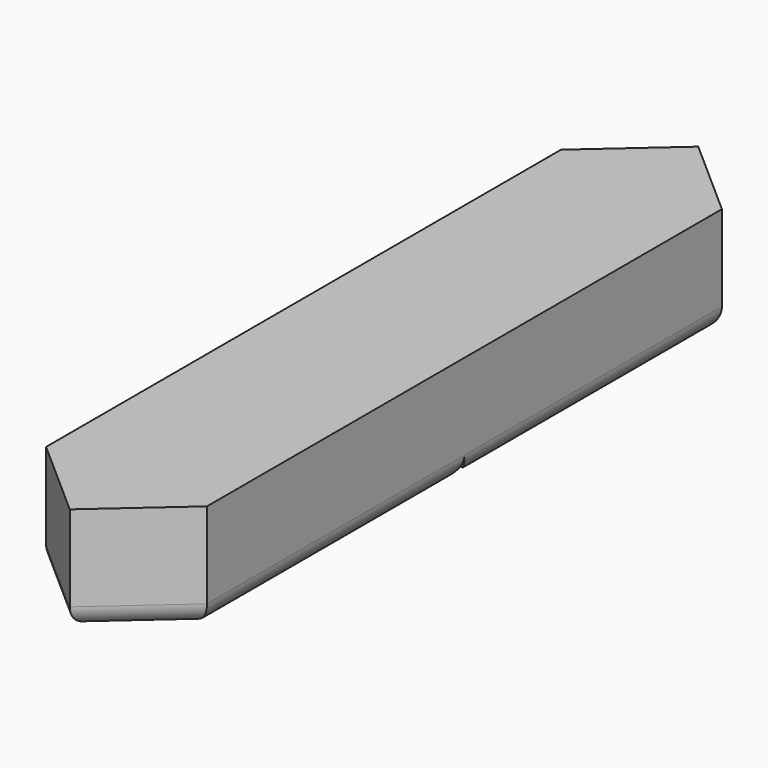
from build123d import *

# Parameters (mm, degrees)
F1_DEPTH    = 25.4
F0_W        = 38.1
F0_H        = 76.2
F2_DEPTH    = 25.4
F3_T        = -2.54
F4_T1_DEPTH = 101.6
F4_T3_DEPTH = 50.8
F4_T5_DEPTH = 50.8
F4_T7_DEPTH = 63.5


# Not quite as in the source:
# - a fillet or chamfer that OpenCascade refuses, or shapes differently, is made with other operations: its cross-section is extruded or revolved along the edge and cut away or added


with BuildPart() as f1:
    # F0 (on Top) → F1 (new body)
    with BuildSketch(Plane.XY):
        Polygon((25.0072174214, -22.3877525396), (-13.0927825786, -22.3877525396), (5.9572174214, -39.1882733649), align=None)
    extrude(amount=F1_DEPTH)

    # F0 (on Top) → F2 (join)
    with BuildSketch(Plane.XY):
        with Locations((5.9572174214, 15.7122474604)):
            Rectangle(F0_W, F0_H)
    extrude(amount=F2_DEPTH)

    # F3
    f3_openings = [f1.faces().sort_by_distance(p)[0] for p in [
        (5.957217, 11.373102, 0),
    ]]
    offset(amount=F3_T, openings=f3_openings)

    # F4: fillet of radius 5.08 on 5 edges, made by hand

    # F4_s2 → F4_t1 (cut)
    with BuildSketch(Plane.XZ.offset(-66.5122474604)):
        with BuildLine():
            ThreePointArc((25.0072174214, 5.08), (23.5193198698, 1.4878975516), (19.9272174214, 0))
            Line((19.9272174214, 0), (25.0072174214, 0))
            Line((25.0072174214, 0), (25.0072174214, 5.08))
        make_face()
        with BuildLine():
            ThreePointArc((-13.0927825786, 5.08), (-11.604885027, 1.4878975516), (-8.0127825786, 0))
            Line((-8.0127825786, 0), (-13.0927825786, 0))
            Line((-13.0927825786, 0), (-13.0927825786, 5.08))
        make_face()
    extrude(amount=F4_T1_DEPTH, mode=Mode.SUBTRACT)

    # F4_s4 → F4_t3 (cut)
    with BuildSketch(Plane(origin=(-25.6145200068, -22.5898832967, 0), x_dir=(0, 0, 1), z_dir=(0.75, 0.6614378278, 0))):
        with BuildLine():
            ThreePointArc((5.08, 33.3315339744), (1.4878975516, 31.8436364228), (0, 28.2515339744))
            Line((0, 28.2515339744), (0, 33.3315339744))
            Line((0, 33.3315339744), (5.08, 33.3315339744))
        make_face()
    extrude(amount=F4_T3_DEPTH, mode=Mode.SUBTRACT)

    # F4_s6 → F4_t5 (cut)
    with BuildSketch(Plane(origin=(-5.7836103942, 5.1006649277, 0), x_dir=(0, 0, 1), z_dir=(0.75, -0.6614378278, 0))):
        with BuildLine():
            ThreePointArc((5.08, 25.4508760729), (1.4878975516, 23.9629785214), (0, 20.3708760729))
            Line((0, 20.3708760729), (0, 25.4508760729))
            Line((0, 25.4508760729), (5.08, 25.4508760729))
        make_face()
    extrude(amount=F4_T5_DEPTH, mode=Mode.SUBTRACT)

    # F4_s8 → F4_t7 (cut)
    with BuildSketch(Plane.YZ.offset(-25.7927825786)):
        with BuildLine():
            ThreePointArc((53.8122474604, 5.08), (52.3243499088, 1.4878975516), (48.7322474604, 0))
            Line((48.7322474604, 0), (53.8122474604, 0))
            Line((53.8122474604, 0), (53.8122474604, 5.08))
        make_face()
    extrude(amount=F4_T7_DEPTH, mode=Mode.SUBTRACT)

    # F5: F1 across face


with BuildPart() as f1_1:
    add(f1.part)
    add(f1.part.mirror(Plane(origin=(5.9572174214, 53.8122474604, 15.24), x_dir=(-1, 0, 0), z_dir=(0, 1, 0))))


solid = f1_1.part
